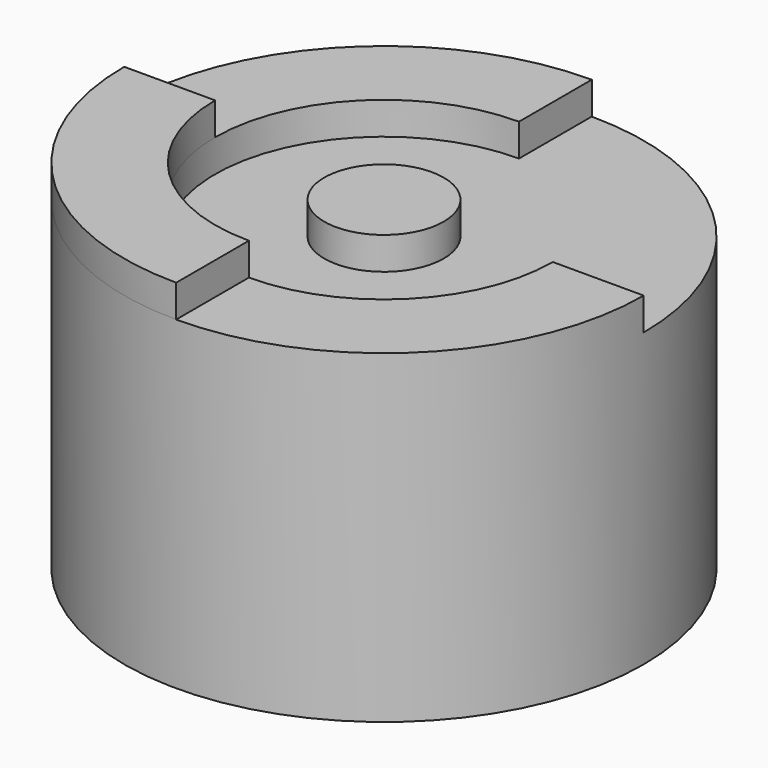
from build123d import *

# Parameters (mm, degrees)
F0_R      = 12.7
F0_R_2    = 8.255
F0_R_3    = 2.921
F1_DEPTH  = 15.875
F2_R      = 8.255
F2_R_2    = 2.921
F3_DEPTH  = 1.5875
F5_DEPTH  = 1.5875
F7_DEPTH  = 1.5875
F9_R      = 10.795
F9_R_2    = 8.255
F10_DEPTH = 9.525
F11_R     = 4.0925147824
F11_R_2   = 2.147201803
F12_DEPTH = 9.525


with BuildPart() as f1:
    # F0 (on Top) → F1 (new body)
    with BuildSketch(Plane.XY):
        Circle(F0_R)
        Circle(F0_R_2, mode=Mode.SUBTRACT)
        Circle(F0_R_2)
        Circle(F0_R_3, mode=Mode.SUBTRACT)
        Circle(F0_R_3)
    extrude(amount=F1_DEPTH)

    # F2 (on face) → F3 (cut)
    with BuildSketch(Plane.XY.offset(15.875)):
        Circle(F2_R)
        Circle(F2_R_2, mode=Mode.SUBTRACT)
    extrude(amount=-F3_DEPTH, mode=Mode.SUBTRACT)

    # F4 (on face) → F5 (cut, through all)
    with BuildSketch(Plane.XY.offset(15.875)):
        with BuildLine():
            ThreePointArc((0, 8.255), (5.8371664787, 5.8371664787), (8.255, 0))
            Line((8.255, 0), (12.7, 0))
            ThreePointArc((12.7, 0), (8.9802561211, 8.9802561211), (0, 12.7))
            Line((0, 12.7), (0, 8.255))
        make_face()
    extrude(amount=-F5_DEPTH, mode=Mode.SUBTRACT)

    # F6 (on face) → F7 (join)
    with BuildSketch(Plane.XY.offset(15.875)):
        with BuildLine():
            Line((0, -12.7), (0, -8.255))
            ThreePointArc((0, -8.255), (-5.8371664787, -5.8371664787), (-8.255, 0))
            Line((-8.255, 0), (-12.7, 0))
            ThreePointArc((-12.7, 0), (-8.9802561211, -8.9802561211), (0, -12.7))
        make_face()
    extrude(amount=F7_DEPTH)

    # F9 (on offset) → F10 (cut)
    with BuildSketch(Plane.XY.offset(2.54)):
        Circle(F9_R)
        Circle(F9_R_2, mode=Mode.SUBTRACT)
    extrude(amount=F10_DEPTH, mode=Mode.SUBTRACT)

    # F11 (on offset) → F12 (cut)
    with BuildSketch(Plane.XY.offset(2.54)):
        Circle(F11_R)
        Circle(F11_R_2, mode=Mode.SUBTRACT)
    extrude(amount=F12_DEPTH, mode=Mode.SUBTRACT)


solid = f1.part
